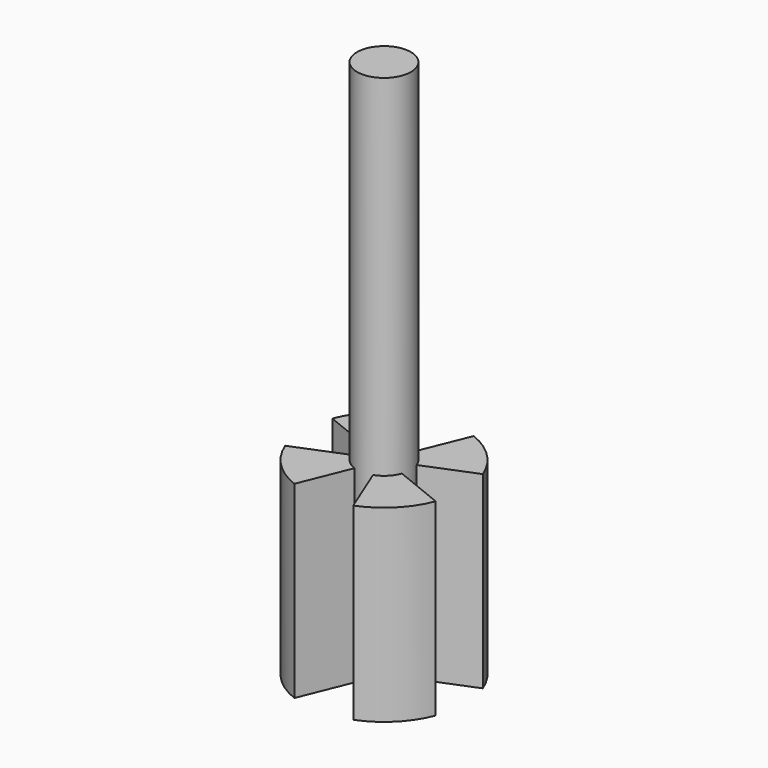
from build123d import *

# Parameters (mm, degrees)
F0_R            = 30
F0_R_2          = 10
F1_DEPTH        = 70
F2_R            = 10
F3_DEPTH        = 130
F3_DEPTH_BACK   = 70
F5_DEPTH        = 70
F5_COPIES_COUNT = 4


# Not quite as in the source:
# - a pattern or mirror of a feature is missing from the dataset's text; its kind, count and spacing are read off the source's solid


with BuildPart() as f1:
    # F0 (on Top) → F1 (new body)
    with BuildSketch(Plane.XY):
        Circle(F0_R)
        Circle(F0_R_2, mode=Mode.SUBTRACT)
    extrude(amount=F1_DEPTH)

    # F2 (on face) → F3 (join, two sides)
    with BuildSketch(Plane.XY.offset(70)) as f3_sk:
        Circle(F2_R)
    extrude(amount=F3_DEPTH)
    extrude(f3_sk.sketch, amount=-F3_DEPTH_BACK)

    # F4 (on face) → F5 (cut, through all)
    with BuildSketch(Plane.XY.offset(70)):
        with BuildLine():
            ThreePointArc((3.4286095737, -9.3938616336), (0, -10), (-3.4286095737, -9.3938616336))
            Line((-3.4286095737, -9.3938616336), (-10.9373596855, -27.9351778786))
            ThreePointArc((-10.9373596855, -27.9351778786), (0, -30), (10.9373596855, -27.9351778786))
            Line((10.9373596855, -27.9351778786), (3.4286095737, -9.3938616336))
        make_face()
    f5 = extrude(amount=-F5_DEPTH, mode=Mode.SUBTRACT)

    # F5_copies: F5 ×4 about axis
    f5_copies_axis = Axis((0, 0, 0), (0, 0, 1))
    for i in range(1, F5_COPIES_COUNT):
        add(f5.rotate(f5_copies_axis, i * 360 / F5_COPIES_COUNT), mode=Mode.SUBTRACT)


solid = f1.part
